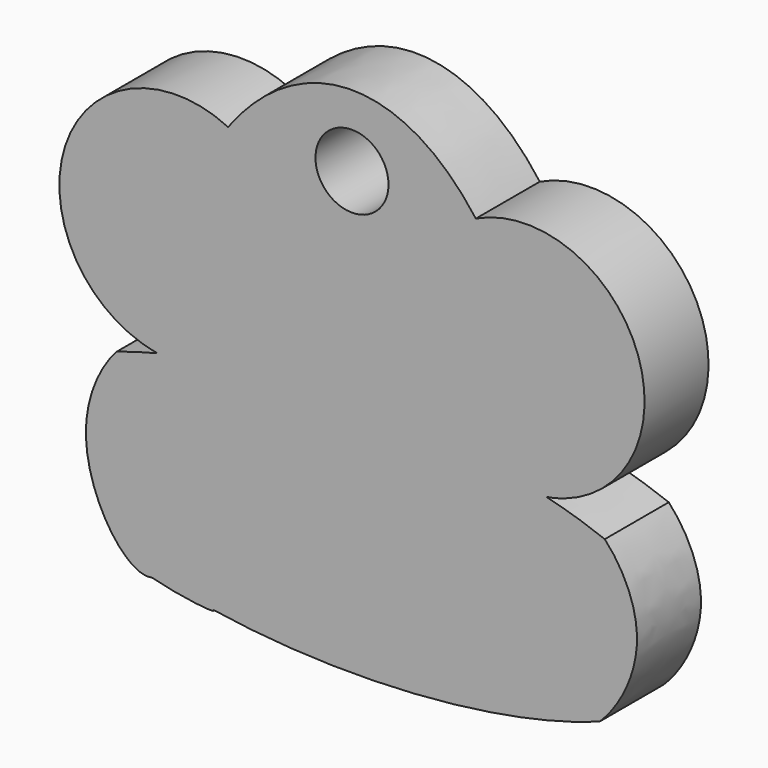
from build123d import *

# Parameters (mm, degrees)
F1_DEPTH = 12.7
F3_DEPTH = 6.35
F5_DEPTH = 6.35
F6_R     = 5.7983245301
F7_DEPTH = 12.7


# Not quite as in the source:
# - a feature names something its author has since deleted; it is built from what else it names


with BuildPart() as f1:
    # F0 (on Front) → F1 (new body)
    with BuildSketch(Plane.XZ):
        with BuildLine():
            add(Edge.make_bspline(
                [(40.1493628068, 1.1925501326), (42.9902625136, -1.8060247086), (47.7076151577, -11.3530425376), (42.6565450289, -21.2863101438), (39.3658101892, -24.5448989348)],
                knots=[0.1578760235, 0.1578760235, 0.1578760235, 0.1578760235, 0.3076794717, 0.476894104, 0.476894104, 0.476894104, 0.476894104], degree=3))
            add(Edge.make_bspline(
                [(40.1493628068, 1.1925501326), (35.9845138771, 2.8298261079), (30.8712290795, 4.0887432654)],
                knots=[0.7315172092, 0.7315172092, 0.7315172092, 0.9616188361, 0.9616188361, 0.9616188361], degree=2, weights=[1, 0.9933889524, 1]))
            add(Edge.make_bspline(
                [(30.8712290795, -27.1396419515), (24.7144737369, -23.1861092597), (24.6668360543, -0.155679542), (30.8712290795, 4.0887432654)],
                knots=[0.6225566131, 0.6225566131, 0.6225566131, 0.6225566131, 1, 1, 1, 1], degree=3))
            add(Edge.make_bspline(
                [(30.8712290795, -27.1396419515), (35.5034035213, -25.9991766513), (39.3658101892, -24.5448989348)],
                knots=[5.3215664711, 5.3215664711, 5.3215664711, 5.530182505, 5.530182505, 5.530182505], degree=2, weights=[1, 0.9945648494, 1]))
        make_face()
        with BuildLine():
            add(Edge.make_bspline(
                [(30.8712290795, -27.1396419515), (24.7144737369, -23.1861092597), (24.6668360543, -0.155679542), (30.8712290795, 4.0887432654)],
                knots=[0.6225566131, 0.6225566131, 0.6225566131, 0.6225566131, 1, 1, 1, 1], degree=3))
            add(Edge.make_bspline(
                [(30.8712290795, 4.0887432654), (0, 11.6893994973), (-30.8712290795, 4.0887432654)],
                knots=[0.9616188361, 0.9616188361, 0.9616188361, 2.1799738175, 2.1799738175, 2.1799738175], degree=2, weights=[1, 0.8201189293, 1]))
            add(Edge.make_bspline(
                [(-30.316427276, -26.6621504769), (-25.7197611969, -21.8642187355), (-25.8183679957, 0.1889268802), (-30.8712290795, 4.0887432654)],
                knots=[0.6258895591, 0.6258895591, 0.6258895591, 0.6258895591, 1, 1, 1, 1], degree=3))
            add(Edge.make_bspline(
                [(-22.0386772722, -28.9035404471), (-22.6123014836, -28.5018760595), (-26.7203664064, -27.4343086812), (-30.316427276, -26.6621504769)],
                knots=[0.351007364, 0.351007364, 0.351007364, 0.351007364, 0.5986156077, 0.5986156077, 0.5986156077, 0.5986156077], degree=3))
            add(Edge.make_bspline(
                [(-22.0386772722, -28.9035404471), (5.8306627498, -33.3047588645), (30.8712290795, -27.1396419515)],
                knots=[4.2915972789, 4.2915972789, 4.2915972789, 5.3215664711, 5.3215664711, 5.3215664711], degree=2, weights=[1, 0.8703003092, 1]))
        make_face()
        with BuildLine():
            add(Edge.make_bspline(
                [(30.8712290795, 4.0887432654), (0, 11.6893994973), (-30.8712290795, 4.0887432654)],
                knots=[0.9616188361, 0.9616188361, 0.9616188361, 2.1799738175, 2.1799738175, 2.1799738175], degree=2, weights=[1, 0.8201189293, 1]))
            add(Edge.make_bspline(
                [(30.8712290795, 4.0887432654), (29.8167825832, 25.6310168931), (19.6674686975, 39.3551867716)],
                knots=[1.651139429, 1.651139429, 1.651139429, 2.4535507775, 2.4535507775, 2.4535507775], degree=2, weights=[1, 0.920590813, 1]))
            add(Edge.make_bspline(
                [(19.6674686975, 39.3551867716), (0, 65.9500565848), (-19.6674686975, 39.3551867716)],
                knots=[2.4535507775, 2.4535507775, 2.4535507775, 3.8296345296, 3.8296345296, 3.8296345296], degree=2, weights=[1, 0.7724909543, 1]))
            add(Edge.make_bspline(
                [(-19.6674686975, 39.3551867716), (-29.8167825832, 25.6310168931), (-30.8712290795, 4.0887432654)],
                knots=[3.8296345296, 3.8296345296, 3.8296345296, 4.6320458782, 4.6320458782, 4.6320458782], degree=2, weights=[1, 0.920590813, 1]))
        make_face()
        with BuildLine():
            add(Edge.make_bspline(
                [(30.8712290795, 4.0887432654), (29.8167825832, 25.6310168931), (19.6674686975, 39.3551867716)],
                knots=[1.651139429, 1.651139429, 1.651139429, 2.4535507775, 2.4535507775, 2.4535507775], degree=2, weights=[1, 0.920590813, 1]))
            add(Edge.make_bspline(
                [(30.8712290795, 4.0887432654), (31.745474043, 4.6868138982), (32.7438524431, 4.9118902663), (33.7979767486, 4.8265914139)],
                knots=[0, 0, 0, 0, 0.0531845708, 0.0531845708, 0.0531845708, 0.0531845708], degree=3))
            ThreePointArc((33.7979767486, 4.8265914139), (45.0771172482, 29.5981627551), (19.6674686975, 39.3551867716))
        make_face()
        with BuildLine():
            add(Edge.make_bspline(
                [(30.8712290795, 4.0887432654), (31.745474043, 4.6868138982), (32.7438524431, 4.9118902663), (33.7979767486, 4.8265914139)],
                knots=[0, 0, 0, 0, 0.0531845708, 0.0531845708, 0.0531845708, 0.0531845708], degree=3))
            ThreePointArc((30.8712290795, 4.0887432654), (32.3495232988, 4.3984841575), (33.7979767486, 4.8265914139))
        make_face()
        with BuildLine():
            add(Edge.make_bspline(
                [(-30.316427276, -26.6621504769), (-25.7197611969, -21.8642187355), (-25.8183679957, 0.1889268802), (-30.8712290795, 4.0887432654)],
                knots=[0.6258895591, 0.6258895591, 0.6258895591, 0.6258895591, 1, 1, 1, 1], degree=3))
            add(Edge.make_bspline(
                [(-30.8712290795, 4.0887432654), (-34.319490328, 3.2397635154), (-37.3534035771, 2.2125195676)],
                knots=[2.1799738175, 2.1799738175, 2.1799738175, 2.335522065, 2.335522065, 2.335522065], degree=2, weights=[1, 0.996977117, 1]))
            add(Edge.make_bspline(
                [(-37.3534035771, 2.2125195676), (-39.9565279998, -0.5633337342), (-46.0541036061, -13.7787361602), (-36.0664526702, -28.5369114032), (-31.8118056749, -27.5574924828)],
                knots=[0.1353541067, 0.1353541067, 0.1353541067, 0.1353541067, 0.2971739822, 0.5889352074, 0.5889352074, 0.5889352074, 0.5889352074], degree=3))
            add(Edge.make_bspline(
                [(-30.316427276, -26.6621504769), (-32.7944749747, -26.1300557959), (-38.0519143989, -25.2083426228), (-34.6365631834, -26.8036586224), (-31.8118056749, -27.5574924828)],
                knots=[0.5986156077, 0.5986156077, 0.5986156077, 0.5986156077, 0.7692425968, 1, 1, 1, 1], degree=3))
        make_face()
        with BuildLine():
            add(Edge.make_bspline(
                [(-30.8712290795, 4.0887432654), (-31.6240605241, 4.6697812862), (-32.4868682621, 4.8478452679), (-33.3934643409, 4.6941488206)],
                knots=[0, 0, 0, 0, 0.0557391345, 0.0557391345, 0.0557391345, 0.0557391345], degree=3))
            add(Edge.make_bspline(
                [(-19.6674686975, 39.3551867716), (-29.8167825832, 25.6310168931), (-30.8712290795, 4.0887432654)],
                knots=[3.8296345296, 3.8296345296, 3.8296345296, 4.6320458782, 4.6320458782, 4.6320458782], degree=2, weights=[1, 0.920590813, 1]))
            ThreePointArc((-19.6674686975, 39.3551867716), (-45.1566020526, 29.4007381707), (-33.3934643409, 4.6941488206))
        make_face()
        with BuildLine():
            ThreePointArc((-33.3934643409, 4.6941488206), (-32.1428628623, 4.3476337433), (-30.8712290795, 4.0887432654))
            add(Edge.make_bspline(
                [(-30.8712290795, 4.0887432654), (-31.6240605241, 4.6697812862), (-32.4868682621, 4.8478452679), (-33.3934643409, 4.6941488206)],
                knots=[0, 0, 0, 0, 0.0557391345, 0.0557391345, 0.0557391345, 0.0557391345], degree=3))
        make_face()
        with BuildLine():
            add(Edge.make_bspline(
                [(-22.0386772722, -28.9035404471), (-22.6123014836, -28.5018760595), (-26.7203664064, -27.4343086812), (-30.316427276, -26.6621504769)],
                knots=[0.351007364, 0.351007364, 0.351007364, 0.351007364, 0.5986156077, 0.5986156077, 0.5986156077, 0.5986156077], degree=3))
            add(Edge.make_bspline(
                [(-31.8118056749, -27.5574924828), (-31.4840598446, -27.4820454557), (-30.9663386258, -27.2558139926), (-30.4943329872, -26.8478458143), (-30.316427276, -26.6621504769)],
                knots=[0.5889352074, 0.5889352074, 0.5889352074, 0.5889352074, 0.6114102859, 0.6258895591, 0.6258895591, 0.6258895591, 0.6258895591], degree=3))
            add(Edge.make_bspline(
                [(-31.8118056749, -27.5574924828), (-27.5150391443, -28.7041566093), (-21.2255124143, -29.4729365051), (-22.0386772722, -28.9035404471)],
                knots=[0, 0, 0, 0, 0.351007364, 0.351007364, 0.351007364, 0.351007364], degree=3))
        make_face()
        with BuildLine():
            add(Edge.make_bspline(
                [(-31.8118056749, -27.5574924828), (-31.4840598446, -27.4820454557), (-30.9663386258, -27.2558139926), (-30.4943329872, -26.8478458143), (-30.316427276, -26.6621504769)],
                knots=[0.5889352074, 0.5889352074, 0.5889352074, 0.5889352074, 0.6114102859, 0.6258895591, 0.6258895591, 0.6258895591, 0.6258895591], degree=3))
            add(Edge.make_bspline(
                [(-30.316427276, -26.6621504769), (-32.7944749747, -26.1300557959), (-38.0519143989, -25.2083426228), (-34.6365631834, -26.8036586224), (-31.8118056749, -27.5574924828)],
                knots=[0.5986156077, 0.5986156077, 0.5986156077, 0.5986156077, 0.7692425968, 1, 1, 1, 1], degree=3))
        make_face()
    extrude(amount=F1_DEPTH)

    # F2 (on Front) → F3 (cut)
    with BuildSketch(Plane.XZ):
        with BuildLine():
            Line((-31.4306877553, 10.459586978), (-23.0095088482, 34.4950370491))
            add(Edge.make_bspline(
                [(-23.0095088482, 34.4950370491), (-25.8661962885, 38.8630829165), (-45.0005379548, 32.5188186692), (-36.4615387565, 9.6457820973), (-31.4306877553, 10.459586978)],
                knots=[0, 0, 0, 0, 0.2940527748, 0.6248688178, 0.6248688178, 0.6248688178, 0.6248688178], degree=3))
        make_face()
        with BuildLine():
            add(Edge.make_bspline(
                [(-13.5356802493, 9.2314984649), (-2.8277460367, 9.2314984649), (-8.181713143, 23.9685634151), (-13.5356802493, 38.7056283653), (-18.8896473556, 23.9685634151), (-24.2436144619, 9.2314984649), (-13.5356802493, 9.2314984649)],
                knots=[0, 0, 0, 2.0943951024, 2.0943951024, 4.1887902048, 4.1887902048, 6.2831853072, 6.2831853072, 6.2831853072], degree=2, weights=[1, 0.5, 1, 0.5, 1, 0.5, 1]))
        make_face()
        with BuildLine():
            add(Edge.make_bspline(
                [(-21.7289508062, -12.611449449), (-21.7321865207, -12.5803032561), (-21.7163109163, -10.9862071439), (-11.1745113639, -14.6318470824), (0, -13.9267453924)],
                knots=[0.7618847301, 0.7618847301, 0.7618847301, 0.7618847301, 0.7662818157, 1, 1, 1, 1], degree=3))
            add(Edge.make_bspline(
                [(0, -13.9267453924), (-12.3324538091, -13.1485785679), (-30.5801397036, -4.9477572556), (-24.4648668208, -10.7903922273), (-21.7289508062, -12.611449449)],
                knots=[0, 0, 0, 0, 0.2579368903, 0.3528249437, 0.3528249437, 0.3528249437, 0.3528249437], degree=3))
        make_face()
        with BuildLine():
            add(Edge.make_bspline(
                [(0, -13.9267453924), (12.3324538091, -13.1485785679), (30.5801396984, -4.9477572579), (24.4648668243, -10.790392224), (21.7289508149, -12.6114494432)],
                knots=[0, 0, 0, 0, 0.2579368903, 0.3528249436, 0.3528249436, 0.3528249436, 0.3528249436], degree=3))
            add(Edge.make_bspline(
                [(21.7289508074, -12.6114494375), (21.7321865206, -12.5803032489), (21.7163108924, -10.9862071522), (11.1745113639, -14.6318470824), (0, -13.9267453924)],
                knots=[0.7618847306, 0.7618847306, 0.7618847306, 0.7618847306, 0.7662818157, 1, 1, 1, 1], degree=3))
        make_face()
        with BuildLine():
            add(Edge.make_bspline(
                [(21.7289508074, -12.6114494375), (21.7321865206, -12.5803032489), (21.7163108924, -10.9862071522), (11.1745113639, -14.6318470824), (0, -13.9267453924)],
                knots=[0.7618847306, 0.7618847306, 0.7618847306, 0.7618847306, 0.7662818157, 1, 1, 1, 1], degree=3))
            add(Edge.make_bspline(
                [(-21.7289508062, -12.611449449), (-21.7321865207, -12.5803032561), (-21.7163109163, -10.9862071439), (-11.1745113639, -14.6318470824), (0, -13.9267453924)],
                knots=[0.7618847301, 0.7618847301, 0.7618847301, 0.7618847301, 0.7662818157, 1, 1, 1, 1], degree=3))
            add(Edge.make_bspline(
                [(-21.7289508062, -12.611449449), (-16.7514821777, -15.9245099169), (-8.1619923275, -20.0642127089), (-3.62e-08, -20.4180739804)],
                knots=[0.3528249437, 0.3528249437, 0.3528249437, 0.3528249437, 0.5254553557, 0.5254553557, 0.5254553557, 0.5254553557], degree=3))
            add(Edge.make_bspline(
                [(21.7289508149, -12.6114494432), (16.7514821877, -15.9245099121), (8.1619922942, -20.064212727), (-3.62e-08, -20.4180739836)],
                knots=[0.3528249436, 0.3528249436, 0.3528249436, 0.3528249436, 0.5254553557, 0.5254553557, 0.5254553557, 0.5254553557], degree=3))
        make_face()
        with BuildLine():
            add(Edge.make_bspline(
                [(23.0095088482, 34.4950370491), (25.8661962885, 38.8630829165), (45.0005379548, 32.5188186692), (36.4615387565, 9.6457820973), (31.4306877553, 10.459586978)],
                knots=[0, 0, 0, 0, 0.2940527748, 0.6248688178, 0.6248688178, 0.6248688178, 0.6248688178], degree=3))
            Line((23.0095088482, 34.4950370491), (31.4306877553, 10.459586978))
        make_face()
        with BuildLine():
            add(Edge.make_bspline(
                [(13.5356802493, 9.2314984649), (24.2436144619, 9.2314984649), (18.8896473556, 23.9685634151), (13.5356802493, 38.7056283653), (8.181713143, 23.9685634151), (2.8277460367, 9.2314984649), (13.5356802493, 9.2314984649)],
                knots=[0, 0, 0, 2.0943951024, 2.0943951024, 4.1887902048, 4.1887902048, 6.2831853072, 6.2831853072, 6.2831853072], degree=2, weights=[1, 0.5, 1, 0.5, 1, 0.5, 1]))
        make_face()
        with BuildLine():
            add(Edge.make_bspline(
                [(-6.7399754189, 0), (-6.7399754189, -1.9063044273), (-3.5605162848, -0.9531522136), (-0.3810571507, 0), (-3.5605162848, 0.9531522136), (-6.7399754189, 1.9063044273), (-6.7399754189, 0)],
                knots=[0, 0, 0, 2.0943951024, 2.0943951024, 4.1887902048, 4.1887902048, 6.2831853072, 6.2831853072, 6.2831853072], degree=2, weights=[1, 0.5, 1, 0.5, 1, 0.5, 1]))
        make_face()
        with BuildLine():
            add(Edge.make_bspline(
                [(6.7399754189, 0), (6.7399754189, 1.9063044273), (3.5605162848, 0.9531522136), (0.3810571507, 0), (3.5605162848, -0.9531522136), (6.7399754189, -1.9063044273), (6.7399754189, 0)],
                knots=[0, 0, 0, 2.0943951024, 2.0943951024, 4.1887902048, 4.1887902048, 6.2831853072, 6.2831853072, 6.2831853072], degree=2, weights=[1, 0.5, 1, 0.5, 1, 0.5, 1]))
        make_face()
    extrude(amount=F3_DEPTH, mode=Mode.SUBTRACT)

    # F6 (on Front) → F7 (cut)
    with BuildSketch(Plane.XZ):
        with Locations((0, 39.5874120295)):
            Circle(F6_R)
    extrude(amount=F7_DEPTH, mode=Mode.SUBTRACT)


with BuildPart() as f5:
    # F4 (on face) → F5 (new body)
    with BuildSketch(Plane(origin=(0, 0, 0), x_dir=(-1, 0, 0), z_dir=(0, 1, 0))):
        with BuildLine():
            add(Edge.make_bspline(
                [(-13.5356802493, 13.6642474681), (-10.5150010112, 13.6642474681), (-12.0253406303, 21.7521889135), (-13.5356802493, 29.8401303589), (-15.0460198684, 21.7521889135), (-16.5563594875, 13.6642474681), (-13.5356802493, 13.6642474681)],
                knots=[0, 0, 0, 2.0943951024, 2.0943951024, 4.1887902048, 4.1887902048, 6.2831853072, 6.2831853072, 6.2831853072], degree=2, weights=[1, 0.5, 1, 0.5, 1, 0.5, 1]))
        make_face()
    extrude(amount=-F5_DEPTH)


with BuildPart() as f5b:
    # F4 (on face) → F5, piece 2 (new body)
    with BuildSketch(Plane(origin=(0, 0, 0), x_dir=(-1, 0, 0), z_dir=(0, 1, 0))):
        with BuildLine():
            add(Edge.make_bspline(
                [(13.5356802493, 13.6642474681), (16.5563594875, 13.6642474681), (15.0460198684, 21.7521889135), (13.5356802493, 29.8401303589), (12.0253406303, 21.7521889135), (10.5150010112, 13.6642474681), (13.5356802493, 13.6642474681)],
                knots=[0, 0, 0, 2.0943951024, 2.0943951024, 4.1887902048, 4.1887902048, 6.2831853072, 6.2831853072, 6.2831853072], degree=2, weights=[1, 0.5, 1, 0.5, 1, 0.5, 1]))
        make_face()
    extrude(amount=-F5_DEPTH)


solid = Compound([f1.part, f5.part, f5b.part])
